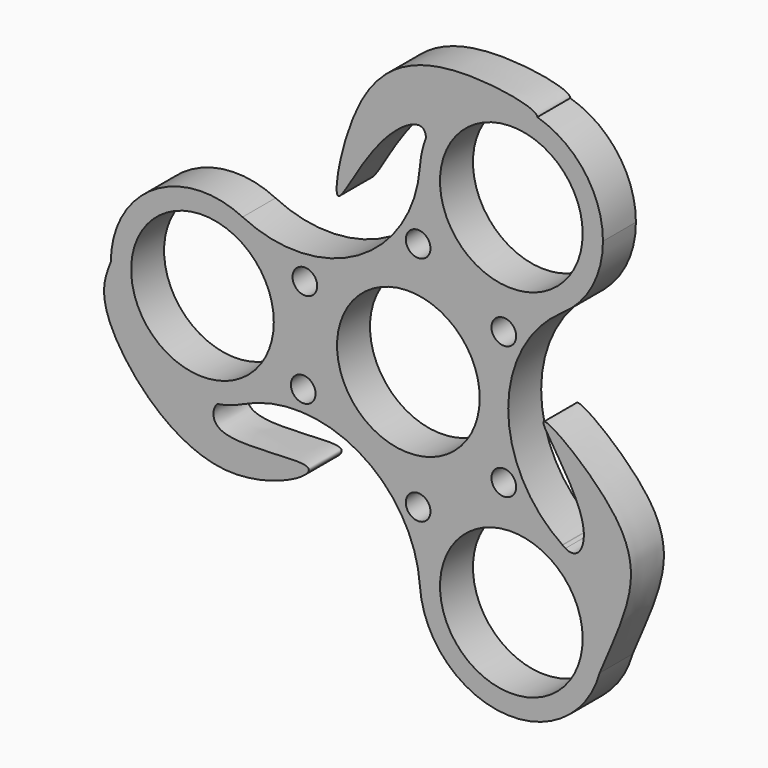
from build123d import *

# Parameters (mm, degrees)
F3_R     = 10.9982
F3_R_2   = 1.905
F3_R_3   = 14.2875
F4_DEPTH = 6.35
F5_R     = 14.2875
F5_R_2   = 10.9982
F6_DEPTH = 6.35


# Not quite as in the source:
# - the dataset's text gives a spline's control points without its knots; the knots are read off the source's solid


with BuildPart() as f4:
    # F3 (on Front) → F4 (new body)
    with BuildSketch(Plane.XZ):
        with BuildLine():
            ThreePointArc((-29.4995777267, -13.9483753948), (-27.48566813, -13.4698570989), (-25.5632910173, -12.7022127413))
            ThreePointArc((-25.5632910173, -12.7022127413), (-17.62125, 0), (-25.5632910173, 12.7022127413))
            ThreePointArc((-25.5632910173, 12.7022127413), (-39.2403642109, 11.9798172169), (-45.87875, 0))
            ThreePointArc((-45.87875, 0), (-40.9104018162, -10.7567939056), (-29.4995777267, -13.9483753948))
        make_face()
        with Locations((-31.75, 0)):
            Circle(F3_R, mode=Mode.SUBTRACT)
        with BuildLine():
            ThreePointArc((-25.5632910173, 12.7022127413), (-17.62125, 0), (-25.5632910173, -12.7022127413))
            ThreePointArc((-25.5632910173, -12.7022127413), (-7.6966609282, -13.3310077763), (1.7812065904, -28.4895657959))
            ThreePointArc((1.7812065904, -28.4895657959), (8.7879219989, -15.2735858432), (23.7385559822, -15.7580757036))
            add(Edge.make_bspline(
                [(23.7370522886, -15.7568490486), (23.7375535577, -15.7572581472), (23.738054789, -15.7576670322), (23.7385559822, -15.7580757036)],
                knots=[0, 0, 0, 0, 2.95195e-05, 2.95195e-05, 2.95195e-05, 2.95195e-05], degree=3))
            ThreePointArc((23.7370522886, -15.7568490486), (15.3933412684, 0.0271955321), (23.7820844269, 15.7873530546))
            ThreePointArc((23.7820844269, 15.7873530546), (8.810625, 15.2604501464), (1.7812065904, 28.4895657959))
            ThreePointArc((1.7812065904, 28.4895657959), (-7.6966609282, 13.3310077763), (-25.5632910173, 12.7022127413))
        make_face()
        with Locations((-16.2175665403, -7.6264850936)):
            Circle(F3_R_2, mode=Mode.SUBTRACT)
        with Locations((1.5040534375, -17.8580671583)):
            Circle(F3_R_2, mode=Mode.SUBTRACT)
        Circle(F3_R_3, mode=Mode.SUBTRACT)
        with Locations((14.7135131028, -10.2315820647)):
            Circle(F3_R_2, mode=Mode.SUBTRACT)
        with Locations((-15.961915625, 7.0821010887)):
            Circle(F3_R_2, mode=Mode.SUBTRACT)
        with Locations((1.5040534375, 17.8580671583)):
            Circle(F3_R_2, mode=Mode.SUBTRACT)
        with Locations((14.7135131028, 10.2315820647)):
            Circle(F3_R_2, mode=Mode.SUBTRACT)
        with BuildLine():
            ThreePointArc((23.7385559822, -15.7580757036), (8.7879219989, -15.2735858432), (1.7812065904, -28.4895657959))
            ThreePointArc((1.7812065904, -28.4895657959), (14.4551677718, -41.5535343554), (29.4855152236, -31.287803888))
            ThreePointArc((29.4855152236, -31.287803888), (29.8735917779, -29.4096818074), (30.00375, -27.4963065702))
            ThreePointArc((30.00375, -27.4963065702), (28.4714616461, -21.097030786), (24.2069554412, -16.085780943))
            add(Edge.make_bspline(
                [(23.7385559822, -15.7580757036), (23.898716393, -15.8886699856), (24.054999522, -15.9974507965), (24.2069554412, -16.085780943)],
                knots=[2.95195e-05, 2.95195e-05, 2.95195e-05, 2.95195e-05, 0.0094627043, 0.0094627043, 0.0094627043, 0.0094627043], degree=3))
        make_face()
        with Locations((15.875, -27.4963065702)):
            Circle(F3_R, mode=Mode.SUBTRACT)
        with BuildLine():
            add(Edge.make_bspline(
                [(-29.4995777267, -13.9483753948), (-30.2603707831, -14.8531192704), (-30.6708700924, -19.7864674308), (-7.0843174646, -15.1494088867), (-31.3734397865, -28.3381470107), (-48.6816596016, -7.9740836174), (-46.7409523482, -2.093253633), (-45.87875, 0)],
                knots=[0.1103018929, 0.1103018929, 0.1103018929, 0.1103018929, 0.2080566397, 0.4028480004, 0.5986420088, 0.8564197656, 1, 1, 1, 1], degree=3))
            ThreePointArc((-29.4995777267, -13.9483753948), (-40.9104018162, -10.7567939056), (-45.87875, 0))
        make_face()
        with BuildLine():
            ThreePointArc((2.7154715941, 32.6391062647), (2.0912937125, 30.5996946449), (1.7812065904, 28.4895657959))
            ThreePointArc((1.7812065904, 28.4895657959), (8.810625, 15.2604501464), (23.7820844269, 15.7873530546))
            ThreePointArc((23.7820844269, 15.7873530546), (28.3517542987, 20.866662633), (30.00375, 27.4963065702))
            ThreePointArc((30.00375, 27.4963065702), (27.1948389939, 35.9510579985), (19.8849749188, 41.0440620194))
            ThreePointArc((19.8849749188, 41.0440620194), (9.6629630907, 40.1861518805), (2.7154715941, 32.6391062647))
        make_face()
        with Locations((15.875, 27.4963065702)):
            Circle(F3_R, mode=Mode.SUBTRACT)
        with BuildLine():
            add(Edge.make_bspline(
                [(23.7370522886, -15.7568490486), (23.7375535577, -15.7572581472), (23.738054789, -15.7576670322), (23.7385559822, -15.7580757036)],
                knots=[0, 0, 0, 0, 2.95195e-05, 2.95195e-05, 2.95195e-05, 2.95195e-05], degree=3))
            ThreePointArc((23.7385559822, -15.7580757036), (23.7603337925, -15.7726941771), (23.7820844269, -15.7873530546))
            ThreePointArc((23.7820844269, -15.7873530546), (23.7595574709, -15.7721171235), (23.7370522886, -15.7568490486))
        make_face()
        with BuildLine():
            ThreePointArc((23.7820844269, -15.7873530546), (23.7603337925, -15.7726941771), (23.7385559822, -15.7580757036))
            add(Edge.make_bspline(
                [(23.7385559822, -15.7580757036), (23.898716393, -15.8886699856), (24.054999522, -15.9974507965), (24.2069554412, -16.085780943)],
                knots=[2.95195e-05, 2.95195e-05, 2.95195e-05, 2.95195e-05, 0.0094627043, 0.0094627043, 0.0094627043, 0.0094627043], degree=3))
            ThreePointArc((24.2069554412, -16.085780943), (23.9958908846, -15.93461518), (23.7820844269, -15.7873530546))
        make_face()
        with BuildLine():
            ThreePointArc((30.00375, -27.4963065702), (29.8735917779, -29.4096818074), (29.4855152236, -31.287803888))
            add(Edge.make_bspline(
                [(24.2069554412, -16.085780943), (26.1006424047, -17.1865583775), (29.6159579428, -11.2149364756), (14.1726228234, 6.181389854), (35.1376160707, -9.4999697108), (34.3521740263, -20.4688665554), (31.4564671012, -26.5945147975), (29.4855152236, -31.287803888)],
                knots=[0.0094627043, 0.0094627043, 0.0094627043, 0.0094627043, 0.1270198173, 0.3477332557, 0.5736567513, 0.7705665051, 0.9611973767, 0.9611973767, 0.9611973767, 0.9611973767], degree=3))
            ThreePointArc((24.2069554412, -16.085780943), (28.4714616461, -21.097030786), (30.00375, -27.4963065702))
        make_face()
        with BuildLine():
            add(Edge.make_bspline(
                [(2.7154715941, 32.6391062647), (2.5583293153, 35.0293568335), (-5.433250301, 31.3542058921), (-13.1618679984, 12.2136359754), (-8.5694718772, 38.2399104562), (5.3216520962, 44.978670844), (19.9201063723, 42.2192816884), (19.8849749188, 41.0440620195)],
                knots=[0.0330162854, 0.0330162854, 0.0330162854, 0.0330162854, 0.1199498348, 0.3181864391, 0.5164230458, 0.7306049733, 0.9133102065, 0.9133102065, 0.9133102065, 0.9133102065], degree=3))
            ThreePointArc((2.7154715941, 32.6391062647), (9.6629630907, 40.1861518805), (19.8849749188, 41.0440620194))
        make_face()
    extrude(amount=F4_DEPTH)

    # F5 (on Front) → F6 (join)
    with BuildSketch(Plane.XZ):
        Circle(F5_R)
        Circle(F5_R_2, mode=Mode.SUBTRACT)
    extrude(amount=F6_DEPTH)


solid = f4.part
